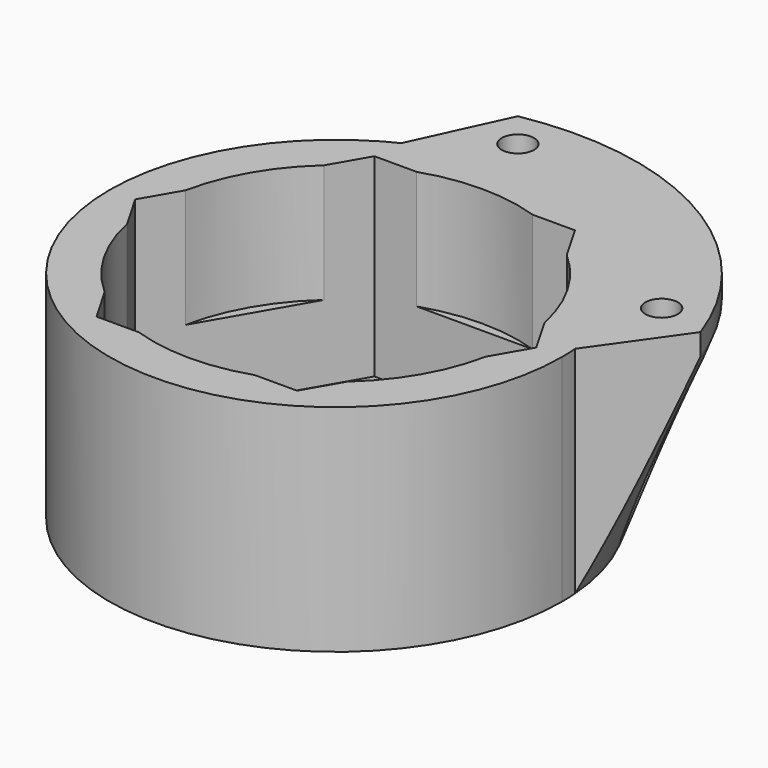
from build123d import *

# Parameters (mm, degrees)
F0_R         = 1.25
F0_R_2       = 5.25
F1_DEPTH     = 2
F2_DEPTH     = 20
F3_DEPTH     = 20
F4_T4_DEPTH  = 68.3486393209
F4_S5_R      = 21
F4_T6_DEPTH  = 36
F4_T10_DEPTH = 68.3486393209
F4_S11_R     = 21
F4_T12_DEPTH = 36
F5_T2_ANGLE  = 272.1691776214
F6_R         = 1.5
F7_DEPTH     = 25
F6_R_2       = 3
F8_DEPTH     = 16
F10_DEPTH    = 11


# Not quite as in the source:
# - a fillet or chamfer that OpenCascade refuses, or shapes differently, is made with other operations: its cross-section is extruded or revolved along the edge and cut away or added


with BuildPart() as f1:
    # F0 (on Top) → F1 (new body)
    with BuildSketch(Plane.XY):
        Polygon((-9.3097730907, -16.125), (9.3097730907, -16.125), (18.6195461814, 0), (9.3097730907, 16.125), (-9.3097730907, 16.125), (-18.6195461814, 0), align=None)
        with Locations((6.982329818, -12.09375)):
            Circle(F0_R, mode=Mode.SUBTRACT)
        with Locations((-13.964659636, 0)):
            Circle(F0_R, mode=Mode.SUBTRACT)
        Circle(F0_R_2, mode=Mode.SUBTRACT)
        with Locations((6.982329818, 12.09375)):
            Circle(F0_R, mode=Mode.SUBTRACT)
    extrude(amount=F1_DEPTH)

    # F0 (on Top) → F2 (join)
    with BuildSketch(Plane.XY):
        with BuildLine():
            ThreePointArc((-10.5, 18.1865334795), (-10.5, -18.1865334795), (21, 0))
            ThreePointArc((21, 0), (10.5, 18.1865334795), (-10.5, 18.1865334795))
        make_face()
        Polygon((18.6195461814, 0), (9.3097730907, -16.125), (-9.3097730907, -16.125), (-18.6195461814, 0), (-9.3097730907, 16.125), (9.3097730907, 16.125), align=None, mode=Mode.SUBTRACT)
    extrude(amount=F2_DEPTH)

    # F0 (on Top) → F3 (join)
    with BuildSketch(Plane.XY):
        with BuildLine():
            ThreePointArc((-10.5, 18.1865334795), (10.5, 18.1865334795), (21, 0))
            Line((21, 0), (28, 0))
            ThreePointArc((28, 0), (14, 24.248711306), (-14, 24.248711306))
            Line((-14, 24.248711306), (-10.5, 18.1865334795))
        make_face()
    extrude(amount=F3_DEPTH)

    # F4: chamfer of 7 on 2 edges, made by hand


with BuildPart() as f4_tool2:
    # F4_s3 → F4_t4 (new body)
    with BuildSketch(Plane.XY.offset(-24.1743196605)):
        with BuildLine():
            Line((-9.8994949366, 17.1464281995), (-5.1164228135, 27.5285709326))
            ThreePointArc((-5.1164228135, 27.5285709326), (-9.6039256501, 26.3014184429), (-14, 24.248711306))
            Line((-14, 24.248711306), (-9.8994949366, 17.1464281995))
        make_face()
    extrude(amount=F4_T4_DEPTH)

    # F4_s5 → F4_t6 (cut, symmetric)
    with BuildSketch(Plane.XY.offset(10)):
        Circle(F4_S5_R)
    extrude(amount=F4_T6_DEPTH, both=True, mode=Mode.SUBTRACT)


with BuildPart() as f1_1:
    add(f1.part)

    # F4_t1: cut F4_tool2
    add(f4_tool2.part, mode=Mode.SUBTRACT)


with BuildPart() as f4_tool8:
    # F4_s9 → F4_t10 (new body)
    with BuildSketch(Plane.XY.offset(-24.1743196605)):
        with BuildLine():
            Line((19.7989898732, 0), (26.3986531643, 9.3333333333))
            ThreePointArc((26.3986531643, 9.3333333333), (27.5796593521, 4.8334656324), (28, 0))
            Line((28, 0), (19.7989898732, 0))
        make_face()
    extrude(amount=F4_T10_DEPTH)

    # F4_s11 → F4_t12 (cut, symmetric)
    with BuildSketch(Plane.XY.offset(10)):
        Circle(F4_S11_R)
    extrude(amount=F4_T12_DEPTH, both=True, mode=Mode.SUBTRACT)


with BuildPart() as f1_2:
    add(f1_1.part)

    # F4_t7: cut F4_tool8
    add(f4_tool8.part, mode=Mode.SUBTRACT)

    # F5: chamfer of 18 x 7 on 1 edges, made by hand

    # F5_s1 → F5_t2 (revolve, cut)
    with BuildSketch(Plane(origin=(0, 0, 0), x_dir=(0, 0, 1), z_dir=(-0.9706518309, -0.2404891332, 0))):
        Polygon((18, -28), (0, -21), (0, -28), align=None)
    revolve(axis=Axis((0, 0, 0), (0, 0, 1)), revolution_arc=F5_T2_ANGLE, mode=Mode.SUBTRACT)

    # F6 (on face) → F7 (cut)
    with BuildSketch(Plane.XY):
        with Locations((21.8586163831, 10.5006375909)):
            Circle(F6_R)
        with Locations((-2.3912845495, 24.1318100897)):
            Circle(F6_R)
    extrude(amount=F7_DEPTH, mode=Mode.SUBTRACT)

    # F6 (on face) → F8 (cut)
    with BuildSketch(Plane.XY):
        with Locations((-2.3912845495, 24.1318100897)):
            Circle(F6_R_2)
        with Locations((-2.3912845495, 24.1318100897)):
            Circle(F6_R, mode=Mode.SUBTRACT)
        with Locations((21.8586163831, 10.5006375909)):
            Circle(F6_R_2)
        with Locations((21.8586163831, 10.5006375909)):
            Circle(F6_R, mode=Mode.SUBTRACT)
    extrude(amount=F8_DEPTH, mode=Mode.SUBTRACT)

    # F9 (on face) → F10 (cut)
    with BuildSketch(Plane.XY.offset(20)):
        with BuildLine():
            ThreePointArc((16.6565165694, -3.4000670246), (16.9139111633, -1.7086863843), (17, 0))
            ThreePointArc((17, 0), (16.9139111633, 1.7086863843), (16.6565165694, 3.4000670246))
            Line((16.6565165694, 3.4000670246), (11.2728027026, 12.7249329754))
            ThreePointArc((11.2728027026, 12.7249329754), (8.5, 14.7224318643), (5.3837138668, 16.125))
            Line((5.3837138668, 16.125), (-5.3837138668, 16.125))
            ThreePointArc((-5.3837138668, 16.125), (-8.5, 14.7224318643), (-11.2728027026, 12.7249329754))
            Line((-11.2728027026, 12.7249329754), (-16.6565165694, 3.4000670246))
            ThreePointArc((-16.6565165694, 3.4000670246), (-17, 0), (-16.6565165694, -3.4000670246))
            Line((-16.6565165694, -3.4000670246), (-11.2728027026, -12.7249329754))
            ThreePointArc((-11.2728027026, -12.7249329754), (-8.5, -14.7224318643), (-5.3837138668, -16.125))
            Line((-5.3837138668, -16.125), (5.3837138668, -16.125))
            ThreePointArc((5.3837138668, -16.125), (8.5, -14.7224318643), (11.2728027026, -12.7249329754))
            Line((11.2728027026, -12.7249329754), (16.6565165694, -3.4000670246))
        make_face()
        with BuildLine():
            Line((11.2728027026, 12.7249329754), (16.6565165694, 3.4000670246))
            ThreePointArc((16.6565165694, 3.4000670246), (14.7224318643, 8.5), (11.2728027026, 12.7249329754))
        make_face()
        with BuildLine():
            ThreePointArc((11.2728027026, -12.7249329754), (14.7224318643, -8.5), (16.6565165694, -3.4000670246))
            Line((16.6565165694, -3.4000670246), (11.2728027026, -12.7249329754))
        make_face()
        with BuildLine():
            Line((-5.3837138668, 16.125), (5.3837138668, 16.125))
            ThreePointArc((5.3837138668, 16.125), (0, 17), (-5.3837138668, 16.125))
        make_face()
        with BuildLine():
            ThreePointArc((-5.3837138668, -16.125), (0, -17), (5.3837138668, -16.125))
            Line((5.3837138668, -16.125), (-5.3837138668, -16.125))
        make_face()
        with BuildLine():
            Line((-16.6565165694, 3.4000670246), (-11.2728027026, 12.7249329754))
            ThreePointArc((-11.2728027026, 12.7249329754), (-14.7224318643, 8.5), (-16.6565165694, 3.4000670246))
        make_face()
        with BuildLine():
            ThreePointArc((-16.6565165694, -3.4000670246), (-14.7224318643, -8.5), (-11.2728027026, -12.7249329754))
            Line((-11.2728027026, -12.7249329754), (-16.6565165694, -3.4000670246))
        make_face()
    extrude(amount=-F10_DEPTH, mode=Mode.SUBTRACT)


solid = f1_2.part
